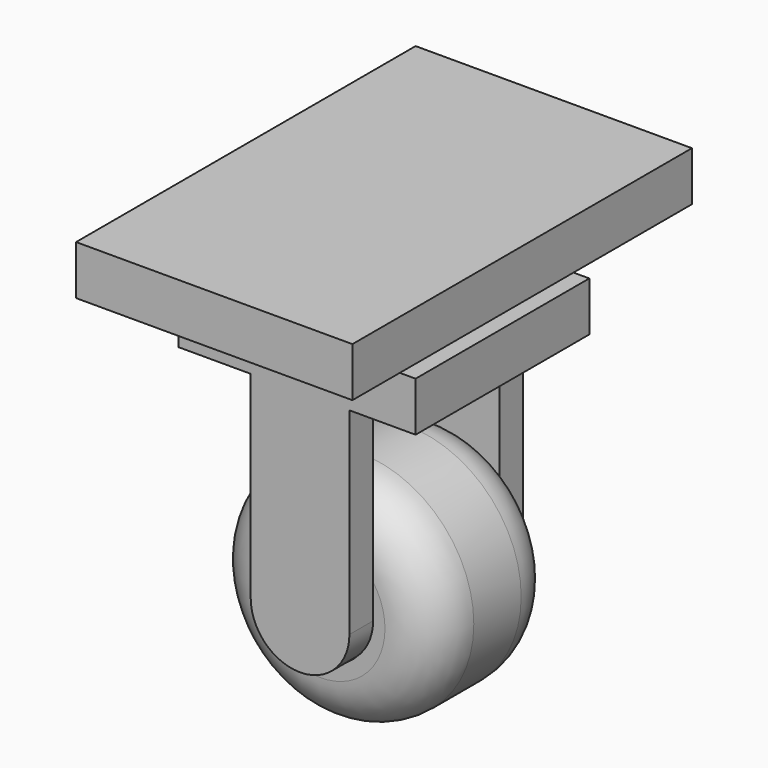
from build123d import *

# Parameters (mm, degrees)
F0_R      = 2.5
F1_DEPTH  = 8
F0_R_2    = 11.5
F0_R_3    = 5
F2_R      = 5
F3_W      = 10
F3_H      = 25
F3_R      = 2.5
F4_DEPTH  = 3
F5_R      = 4.99999
F6_W      = 10
F6_H      = 3
F7_DEPTH  = 5
F8_R      = 2.5
F9_DEPTH  = 3
F10_R     = 5
F11_R     = 9
F12_DEPTH = 3
F13_W     = 28
F13_H     = 43
F13_R     = 9
F14_DEPTH = 5


# Not quite as in the source:
# - a fillet or chamfer is up to 0.001 mm smaller than in the source, because OpenCascade refuses the exact size


with BuildPart() as f1:
    # F0 (on Front) → F1 (new body, symmetric)
    with BuildSketch(Plane.XZ):
        Circle(F0_R)
    extrude(amount=F1_DEPTH, both=True)


with BuildPart() as f1b:
    # F0 (on Front) → F1, piece 2 (new body, symmetric)
    with BuildSketch(Plane.XZ):
        Circle(F0_R_2)
        Circle(F0_R_3, mode=Mode.SUBTRACT)
    extrude(amount=F1_DEPTH, both=True)

    # F2
    f2_edges = [f1b.edges().sort_by_distance(p)[0] for p in [
        (-11.5, 8, 0),
        (11.5, 0, 0),
        (-11.5, -8, 0),
    ]]
    fillet(f2_edges, radius=F2_R)


with BuildPart() as f4:
    # F3 (on face) → F4 (new body)
    with BuildSketch(Plane.XZ.offset(8)):
        with Locations((0.2946209682, 7.8014951967)):
            Rectangle(F3_W, F3_H)
        Circle(F3_R, mode=Mode.SUBTRACT)
        Circle(F3_R)
    extrude(amount=F4_DEPTH)

    # F5 (radius 5 in the source; OpenCascade refuses exactly that, so slightly less here)
    f5_edges = [f4.edges().sort_by_distance(p)[0] for p in [
        (-4.705379, -9.5, -4.698505),
        (5.294621, -9.5, -4.698505),
    ]]
    fillet(f5_edges, radius=F5_R)

    # F6 (on face) → F7 (join)
    with BuildSketch(Plane.XY.offset(20.3014951967)):
        Polygon((5.2946209682, -11), (12, -11), (12, 11), (-12, 11), (-12, -11), (-4.7053790318, -11), (-4.7053790318, -8), (5.2946209682, -8), align=None)
        with Locations((0.2946209682, -9.5)):
            Rectangle(F6_W, F6_H)
    extrude(amount=F7_DEPTH)

    # F11 (on face) → F12 (join)
    with BuildSketch(Plane.XY.offset(25.3014951967)):
        Circle(F11_R)
    extrude(amount=F12_DEPTH)

    # F13 (on face) → F14 (join)
    with BuildSketch(Plane.XY.offset(28.3014951967)):
        Rectangle(F13_W, F13_H)
        Circle(F13_R, mode=Mode.SUBTRACT)
        Circle(F13_R)
    extrude(amount=F14_DEPTH)


with BuildPart() as f9:
    # F8 (on face) → F9 (new body)
    with BuildSketch(Plane(origin=(0, 8, 0), x_dir=(-1, 0, 0), z_dir=(0, 1, 0))):
        Polygon((4.7053790318, 20.3014951967), (-5.2946209908, 20.3014951967), (-5.2946209908, 4.3689608574), (-5.2946209908, -4.3689608574), (4.7053790318, -4.3689608574), (4.7053790318, 4.3689608574), align=None)
        Circle(F8_R, mode=Mode.SUBTRACT)
        Circle(F8_R)
    extrude(amount=F9_DEPTH)

    # F10
    f10_edges = [f9.edges().sort_by_distance(p)[0] for p in [
        (5.294621, 9.5, -4.368961),
        (-4.705379, 9.5, -4.368961),
    ]]
    fillet(f10_edges, radius=F10_R)


solid = Compound([f1.part, f1b.part, f4.part, f9.part])
